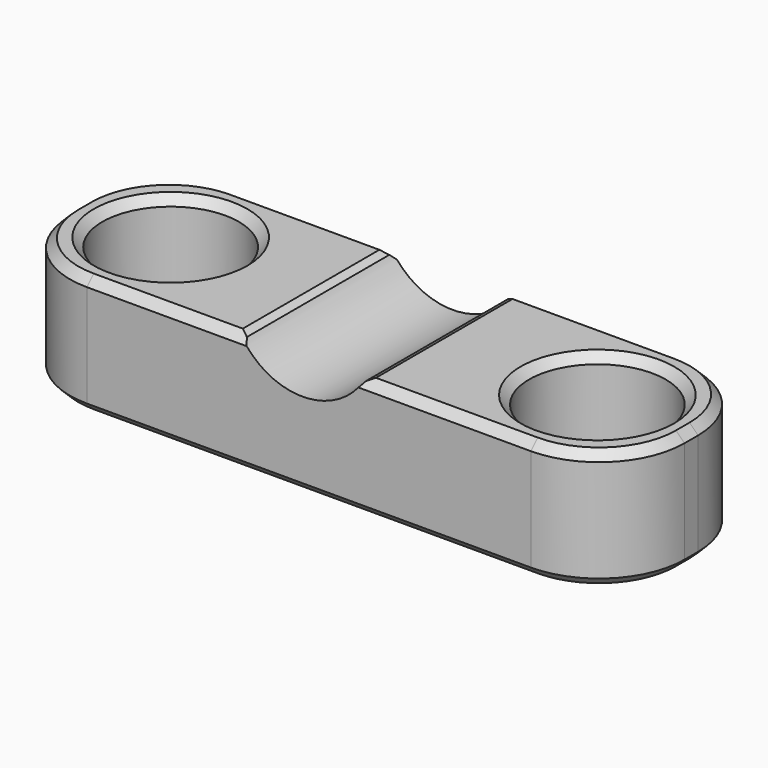
from build123d import *

# Parameters (mm, degrees)
F0_R         = 4
F1_DEPTH     = 7
F3_DEPTH     = 25
F4_T1_DEPTH  = 26
F4_T3_DEPTH  = 1
F4_T5_DEPTH  = 10.285841494
F4_T7_DEPTH  = 12.4424386412
F4_T9_DEPTH  = 11.029084367
F4_T12_ANGLE = 90
F4_T14_ANGLE = 90
F4_T16_ANGLE = 90
F4_T18_ANGLE = 90
F4_T24_ANGLE = 90
F4_T26_ANGLE = 90
F4_T30_ANGLE = 90
F4_T32_ANGLE = 90


# Not quite as in the source:
# - a fillet or chamfer that OpenCascade refuses, or shapes differently, is made with other operations: its cross-section is extruded or revolved along the edge and cut away or added


with BuildPart() as f1:
    # F0 (on Top) → F1 (new body)
    with BuildSketch(Plane.XY):
        with BuildLine():
            Line((25.5, 5.5), (-0.5, 5.5))
            ThreePointArc((-0.5, 5.5), (-4.0355339059, 4.0355339059), (-5.5, 0.5))
            Line((-5.5, 0.5), (-5.5, -0.5))
            ThreePointArc((-5.5, -0.5), (-4.0355339059, -4.0355339059), (-0.5, -5.5))
            Line((-0.5, -5.5), (25.5, -5.5))
            ThreePointArc((25.5, -5.5), (29.0355339059, -4.0355339059), (30.5, -0.5))
            Line((30.5, -0.5), (30.5, 0.5))
            ThreePointArc((30.5, 0.5), (29.0355339059, 4.0355339059), (25.5, 5.5))
        make_face()
        Circle(F0_R, mode=Mode.SUBTRACT)
        with Locations((25, 0)):
            Circle(F0_R, mode=Mode.SUBTRACT)
    extrude(amount=F1_DEPTH)

    # F2 (on face) → F3 (cut)
    with BuildSketch(Plane.XZ.offset(5.5)):
        with BuildLine():
            Line((15.756757127, 7), (8.5, 7))
            ThreePointArc((8.5, 7), (12.1283785635, 4.963), (15.756757127, 7))
        make_face()
    extrude(amount=-F3_DEPTH, mode=Mode.SUBTRACT)

    # F4: chamfer of 0.5 on 24 edges, made by hand

    # F4_s2 → F4_t1 (cut)
    with BuildSketch(Plane.YZ.offset(-0.5)):
        Polygon((-5, 0), (-5.5, 0.5), (-5.5, 0), align=None)
        Polygon((5, 0), (5.5, 0.5), (5.5, 0), align=None)
    extrude(amount=F4_T1_DEPTH, mode=Mode.SUBTRACT)

    # F4_s4 → F4_t3 (cut)
    with BuildSketch(Plane.XZ.offset(-0.5)):
        Polygon((30.5, 0.5), (30, 0), (30.5, 0), align=None)
        Polygon((-5, 0), (-5.5, 0.5), (-5.5, 0), align=None)
        Polygon((-5.5, 6.5), (-5, 7), (-5.5, 7), align=None)
        Polygon((30.5, 6.5), (30, 7), (30.5, 7), align=None)
    extrude(amount=F4_T3_DEPTH, mode=Mode.SUBTRACT)

    # F4_s6 → F4_t5 (cut)
    with BuildSketch(Plane.YZ.offset(-0.5)):
        Polygon((-5.5, 6.5), (-5, 7), (-5.5, 7), align=None)
        Polygon((5.5, 6.5), (5, 7), (5.5, 7), align=None)
    extrude(amount=F4_T5_DEPTH, mode=Mode.SUBTRACT)

    # F4_s8 → F4_t7 (cut)
    with BuildSketch(Plane.XZ.offset(-6.2212193206)):
        with BuildLine():
            Line((8.6398076479, 6.7855789474), (8.2293875402, 7))
            Line((8.2293875402, 7), (8.5, 7))
            ThreePointArc((8.5, 7), (8.5730669131, 6.8844255286), (8.6398076479, 6.7855789474))
        make_face()
        with BuildLine():
            Line((16.0273695868, 7), (15.6169494791, 6.7855789474))
            ThreePointArc((15.6169494791, 6.7855789474), (15.6836902138, 6.8844255286), (15.756757127, 7))
            Line((15.756757127, 7), (16.0273695868, 7))
        make_face()
    extrude(amount=F4_T7_DEPTH, mode=Mode.SUBTRACT)

    # F4_s10 → F4_t9 (cut)
    with BuildSketch(Plane.YZ.offset(14.470915633)):
        Polygon((-5, 7), (-5.5, 6.5), (-5.5, 7), align=None)
        Polygon((5, 7), (5.5, 6.5), (5.5, 7), align=None)
    extrude(amount=F4_T9_DEPTH, mode=Mode.SUBTRACT)

    # F4_s11 → F4_t12 (revolve, cut)
    with BuildSketch(Plane.XZ.offset(-0.5)):
        Polygon((30.5, 0.5), (30, 0), (30.5, 0), align=None)
    revolve(axis=Axis((25.5, 0.5, 0), (0, 0, 1)), revolution_arc=F4_T12_ANGLE, mode=Mode.SUBTRACT)

    # F4_s13 → F4_t14 (revolve, cut)
    with BuildSketch(Plane.YZ.offset(-0.5)):
        Polygon((5, 0), (5.5, 0.5), (5.5, 0), align=None)
    revolve(axis=Axis((-0.5, 0.5, 0), (0, 0, 1)), revolution_arc=F4_T14_ANGLE, mode=Mode.SUBTRACT)

    # F4_s15 → F4_t16 (revolve, cut)
    with BuildSketch(Plane.XZ.offset(0.5)):
        Polygon((-5, 0), (-5.5, 0.5), (-5.5, 0), align=None)
    revolve(axis=Axis((-0.5, -0.5, 0), (0, 0, 1)), revolution_arc=F4_T16_ANGLE, mode=Mode.SUBTRACT)

    # F4_s17 → F4_t18 (revolve, cut)
    with BuildSketch(Plane.YZ.offset(25.5)):
        Polygon((-5.5, 0.5), (-5, 0), (-5.5, 0), align=None)
    revolve(axis=Axis((25.5, -0.5, 0), (0, 0, 1)), revolution_arc=F4_T18_ANGLE, mode=Mode.SUBTRACT)

    # F4_s19 → F4_t20 (revolve, cut)
    with BuildSketch(Plane.XZ):
        Polygon((4.5, 0), (4, 0.5), (4, 0), align=None)
    revolve(axis=Axis((0, 0, 0), (0, 0, 1)), mode=Mode.SUBTRACT)

    # F4_s21 → F4_t22 (revolve, cut)
    with BuildSketch(Plane.XZ):
        Polygon((29.5, 0), (29, 0.5), (29, 0), align=None)
    revolve(axis=Axis((25, 0, 0), (0, 0, 1)), mode=Mode.SUBTRACT)

    # F4_s23 → F4_t24 (revolve, cut)
    with BuildSketch(Plane.XZ.offset(0.5)):
        Polygon((-5.5, 6.5), (-5, 7), (-5.5, 7), align=None)
    revolve(axis=Axis((-0.5, -0.5, 7), (0, 0, 1)), revolution_arc=F4_T24_ANGLE, mode=Mode.SUBTRACT)

    # F4_s25 → F4_t26 (revolve, cut)
    with BuildSketch(Plane.YZ.offset(-0.5)):
        Polygon((5.5, 6.5), (5, 7), (5.5, 7), align=None)
    revolve(axis=Axis((-0.5, 0.5, 7), (0, 0, 1)), revolution_arc=F4_T26_ANGLE, mode=Mode.SUBTRACT)

    # F4_s27 → F4_t28 (revolve, cut)
    with BuildSketch(Plane.XZ):
        Polygon((4, 6.5), (4.5, 7), (4, 7), align=None)
    revolve(axis=Axis((0, 0, 7), (0, 0, 1)), mode=Mode.SUBTRACT)

    # F4_s29 → F4_t30 (revolve, cut)
    with BuildSketch(Plane.YZ.offset(25.5)):
        Polygon((-5.5, 6.5), (-5, 7), (-5.5, 7), align=None)
    revolve(axis=Axis((25.5, -0.5, 7), (0, 0, 1)), revolution_arc=F4_T30_ANGLE, mode=Mode.SUBTRACT)

    # F4_s31 → F4_t32 (revolve, cut)
    with BuildSketch(Plane.XZ.offset(-0.5)):
        Polygon((30.5, 6.5), (30, 7), (30.5, 7), align=None)
    revolve(axis=Axis((25.5, 0.5, 7), (0, 0, 1)), revolution_arc=F4_T32_ANGLE, mode=Mode.SUBTRACT)

    # F4_s33 → F4_t34 (revolve, cut)
    with BuildSketch(Plane.XZ):
        Polygon((29.5, 7), (29, 6.5), (29, 7), align=None)
    revolve(axis=Axis((25, 0, 7), (0, 0, 1)), mode=Mode.SUBTRACT)


solid = f1.part
